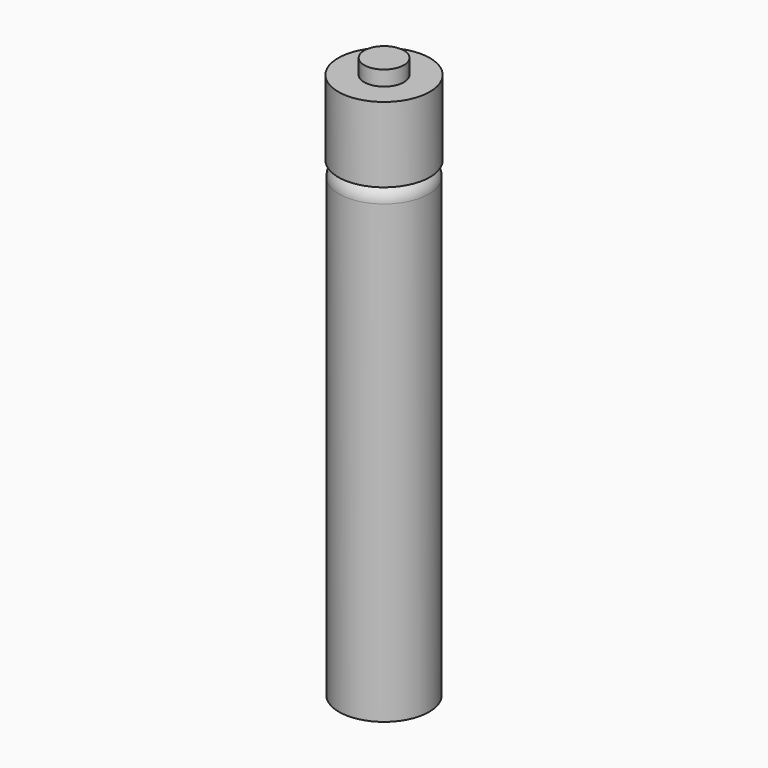
from build123d import *

# Parameters (mm, degrees)
F0_W      = 9
F0_H      = 89
F2_R      = 9
F3_DEPTH  = 5
F4_R      = 3
F5_R      = 7
F6_DEPTH  = 11
F8_DEPTH  = 11
F10_R     = 3.9621233683
F11_DEPTH = 18
F9_R      = 9.1436864808
F12_DEPTH = 15


with BuildPart() as f1:
    # F0 (on Front) → F1 (revolve)
    with BuildSketch(Plane.XZ):
        with Locations((4.5, 44.5)):
            Rectangle(F0_W, F0_H)
    revolve(axis=Axis((0, 0, 44.5), (0, 0, -1)))

    # F2 (on face) → F3 (join)
    with BuildSketch(Plane.XY.offset(89)):
        Circle(F2_R)
    extrude(amount=F3_DEPTH)

    # F4
    f4_edges = [f1.edges().sort_by_distance(p)[0] for p in [
        (-9, 0, 94),
    ]]
    fillet(f4_edges, radius=F4_R)

    # F5 (on face) → F6 (cut)
    with BuildSketch(Plane(origin=(0, 0, 0), x_dir=(1, 0, 0), z_dir=(0, 0, -1))):
        Circle(F5_R)
    extrude(amount=-F6_DEPTH, mode=Mode.SUBTRACT)

    # F7 (on face) → F8 (join)
    with BuildSketch(Plane(origin=(0, 0, 11), x_dir=(1, 0, 0), z_dir=(0, 0, -1))):
        with BuildLine():
            Line((-0.5, 5), (0, 5))
            Line((0, 5), (0.5, 5))
            Line((0.5, 5), (0.5, 6.9821200219))
            ThreePointArc((0.5, 6.9821200219), (0, 7), (-0.5, 6.9821200219))
            Line((-0.5, 6.9821200219), (-0.5, 5))
        make_face()
        with BuildLine():
            ThreePointArc((7, 0), (6.9955285774, 0.2501597957), (6.9821200219, 0.5))
            Line((6.9821200219, 0.5), (5, 0.5))
            Line((5, 0.5), (5, 0))
            Line((5, 0), (5, -0.5))
            Line((5, -0.5), (6.9821200219, -0.5))
            ThreePointArc((6.9821200219, -0.5), (6.9955285774, -0.2501597957), (7, 0))
        make_face()
        with BuildLine():
            Line((-5, 0.5), (-6.9821200219, 0.5))
            ThreePointArc((-6.9821200219, 0.5), (-7, 0), (-6.9821200219, -0.5))
            Line((-6.9821200219, -0.5), (-5, -0.5))
            Line((-5, -0.5), (-5, 0))
            Line((-5, 0), (-5, 0.5))
        make_face()
        with BuildLine():
            Line((-0.5, -5), (-0.5, -6.9821200219))
            ThreePointArc((-0.5, -6.9821200219), (0, -7), (0.5, -6.9821200219))
            Line((0.5, -6.9821200219), (0.5, -5))
            Line((0.5, -5), (0, -5))
            Line((0, -5), (-0.5, -5))
        make_face()
    extrude(amount=F8_DEPTH)

    # F10 (on face) → F11 (join)
    with BuildSketch(Plane.XY.offset(94)):
        Circle(F10_R)
    extrude(amount=F11_DEPTH)

    # F9 (on face) → F12 (join)
    with BuildSketch(Plane.XY.offset(94)):
        Circle(F9_R)
    extrude(amount=F12_DEPTH)


solid = f1.part
